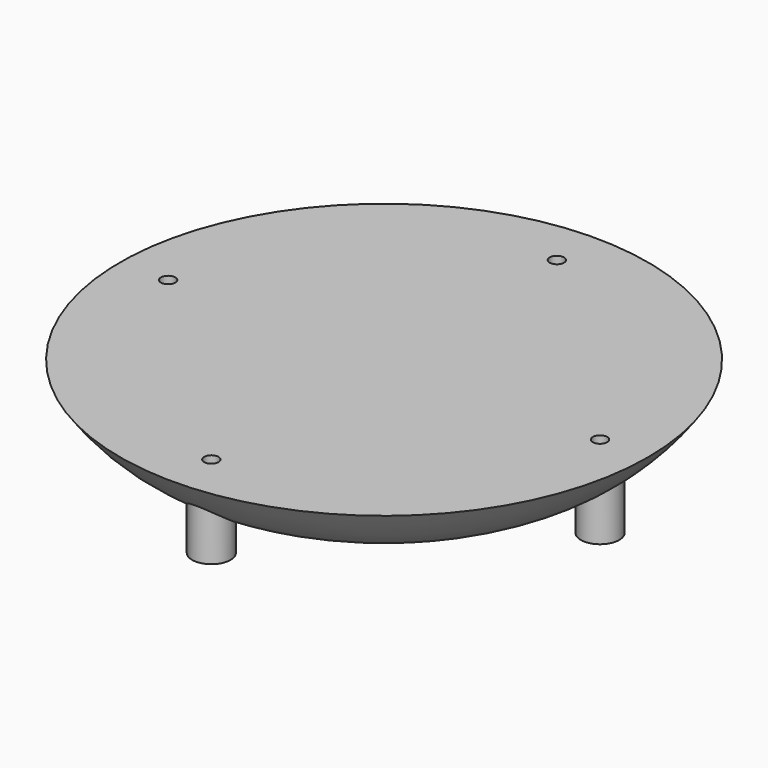
from build123d import *

# Parameters (mm, degrees)
F3_R     = 4
F4_DEPTH = 12
F5_R     = 1.5
F6_DEPTH = 25


with BuildPart() as f1:
    # F0 (on Front) → F1 (revolve)
    with BuildSketch(Plane.XZ):
        with BuildLine():
            Line((0, 19.93), (0, 2.5))
            Line((0, 2.5), (5, 2.5))
            add(Edge.make_bspline(
                [(5, 2.5), (5.3328510826, 2.4217743273), (5.9964782101, 2.2658106511), (6.9983179352, 2.1197039578), (7.9995053084, 2.0366561555), (8.9996417233, 1.9739737746), (9.9999165926, 1.9475438797), (11.0000008446, 1.935865527), (12.0000383829, 1.9489951187), (13.0000622241, 1.9681576208), (14.0000874592, 1.9983838356), (15.0001122592, 2.0383255927), (16.0001370916, 2.0883442574), (17.0001618271, 2.148342783), (18.0001864282, 2.2183478788), (19.0002110875, 2.2983497638), (20.0002349857, 2.3883608236), (21.0002611249, 2.4883412474), (22.0002782257, 2.5984379641), (23.0003283544, 2.7181026114), (24.0002543135, 2.8493833922), (25.000895917, 2.9846630387), (25.9998052646, 3.1525131019), (27.0009227888, 3.3054508496), (28.0009713029, 3.4864375887), (29.0003478858, 3.6897873256), (30.0012434797, 3.8951500576), (31.0002728406, 4.1308468645), (32.0021624026, 4.3625117569), (33.0002529532, 4.6414496195), (34.0023629695, 4.9132136305), (35.0011881909, 5.2289056776), (36.0025557063, 5.5542640629), (37.0014311173, 5.9184670669), (38.0025624421, 6.2958891719), (39.0037946478, 6.7040678184), (40.0028107947, 7.1566870694), (41.0027396353, 7.6374785101), (42.0055454925, 8.1429278876), (43.004228325, 8.7064011364), (44.004224438, 9.306997806), (45.0073247322, 9.9432016714), (46.0057995192, 10.6465378886), (47.0058234103, 11.3970699492), (48.0088937531, 12.1945745949), (49.0086544899, 13.0664036563), (50.0086681154, 14.007093901), (51.009971062, 15.0171879868), (52.0113800481, 16.1070392374), (53.010593298, 17.2897231439), (54.0131863874, 18.5559560931), (54.6684343672, 19.4683264564), (55, 19.93)],
                knots=[0, 0, 0, 0, 0.0192342727, 0.0383486364, 0.0573953442, 0.0764207609, 0.0954333686, 0.1144421761, 0.1334509836, 0.1524612165, 0.1714738242, 0.1904897553, 0.2095099566, 0.2285353734, 0.2475669482, 0.2666056211, 0.285652329, 0.3047080049, 0.3237735783, 0.3428499742, 0.3619381127, 0.3810389089, 0.4001677438, 0.4192965787, 0.4384570424, 0.4576526715, 0.4768671915, 0.4961220706, 0.5153984017, 0.534744074, 0.5541144917, 0.5735639074, 0.5930698576, 0.6126662076, 0.6323264323, 0.6520876645, 0.6719928068, 0.6920124161, 0.7121517577, 0.7325015415, 0.7530286956, 0.7737405025, 0.7947415319, 0.8159934935, 0.837504215, 0.8593884201, 0.8816569315, 0.9043183574, 0.9274369188, 0.9510771906, 0.9752443002, 1, 1, 1, 1], degree=3))
            Line((55, 19.93), (0, 19.93))
        make_face()
    revolve(axis=Axis((0, 0, 5.0231479108), (0, 0, 1)))

    # F3 (on offset) → F4 (join)
    with BuildSketch(Plane.XY.offset(2.8)):
        with Locations((0, -45)):
            Circle(F3_R)
        with Locations((45, 0)):
            Circle(F3_R)
        with Locations((0, 45)):
            Circle(F3_R)
        with Locations((-45, 0)):
            Circle(F3_R)
    extrude(amount=F4_DEPTH)

    # F5 (on offset) → F6 (cut)
    with BuildSketch(Plane.XY.offset(2.8)):
        with Locations((45, 0)):
            Circle(F5_R)
        with Locations((0, -45)):
            Circle(F5_R)
        with Locations((-45, 0)):
            Circle(F5_R)
        with Locations((0, 45)):
            Circle(F5_R)
    extrude(amount=F6_DEPTH, mode=Mode.SUBTRACT)

    # F7 (on Front) → F8 (revolve)
    with BuildSketch(Plane.XZ):
        Polygon((4, 2.5), (0, 2.5), (0, 0.5), align=None)
    revolve(axis=Axis((0, 0, 9.9652772769), (0, 0, 1)))


solid = f1.part
